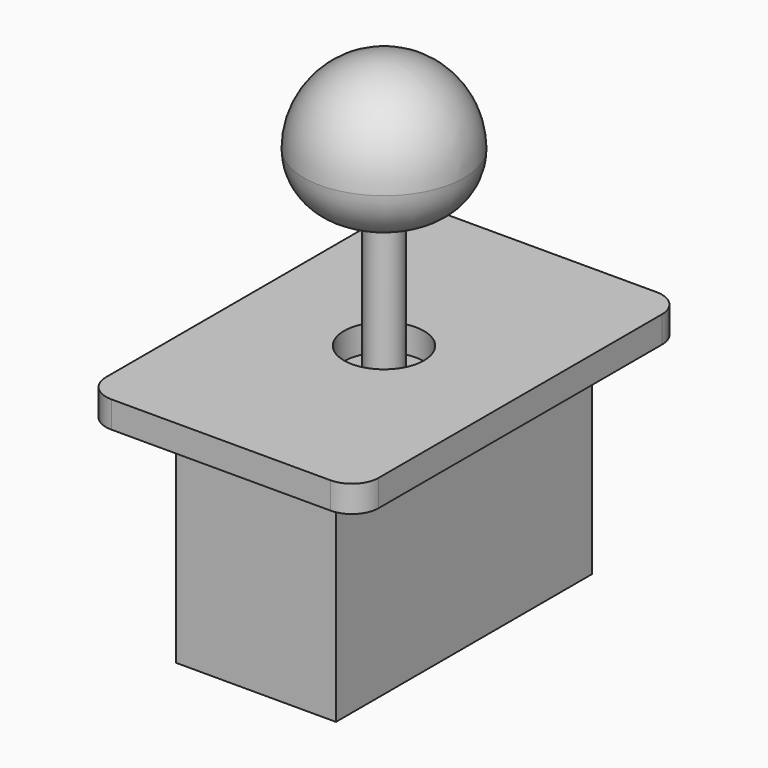
from build123d import *

# Parameters (mm, degrees)
F0_R     = 9.525
F1_DEPTH = 6.35
F2_R     = 4.1191118401
F3_DEPTH = 35
F4_R     = 19.05
F5_DEPTH = 31.75
F6_R     = 19.05
F7_R     = 12.69999
F8_W     = 38.1
F8_H     = 76.2
F8_R     = 9.525
F9_DEPTH = 50.8


# Not quite as in the source:
# - a fillet or chamfer is up to 0.001 mm smaller than in the source, because OpenCascade refuses the exact size


with BuildPart() as f1:
    # F0 (on Top) → F1 (new body)
    with BuildSketch(Plane.XY):
        with BuildLine():
            Line((26.095, 48.505), (-26.095, 48.505))
            ThreePointArc((-26.095, 48.505), (-30.5851280605, 46.6451280605), (-32.445, 42.155))
            Line((-32.445, 42.155), (-32.445, -42.155))
            ThreePointArc((-32.445, -42.155), (-30.5851280605, -46.6451280605), (-26.095, -48.505))
            Line((-26.095, -48.505), (26.095, -48.505))
            ThreePointArc((26.095, -48.505), (30.5851280605, -46.6451280605), (32.445, -42.155))
            Line((32.445, -42.155), (32.445, 42.155))
            ThreePointArc((32.445, 42.155), (30.5851280605, 46.6451280605), (26.095, 48.505))
        make_face()
        Circle(F0_R, mode=Mode.SUBTRACT)
    extrude(amount=-F1_DEPTH)


with BuildPart() as f3:
    # F2 (on face) → F3 (new body)
    with BuildSketch(Plane(origin=(0, 0, -6.35), x_dir=(1, 0, 0), z_dir=(0, 0, -1))):
        Circle(F2_R)
    extrude(amount=-F3_DEPTH)

    # F4 (on face) → F5 (join)
    with BuildSketch(Plane.XY.offset(28.65)):
        Circle(F4_R)
    extrude(amount=F5_DEPTH)

    # F6
    f6_edges = [f3.edges().sort_by_distance(p)[0] for p in [
        (-19.05, 0, 60.4),
    ]]
    fillet(f6_edges, radius=F6_R)

    # F7 (radius 12.7 in the source; OpenCascade refuses exactly that, so slightly less here)
    f7_edges = [f3.edges().sort_by_distance(p)[0] for p in [
        (-19.05, 0, 28.65),
    ]]
    fillet(f7_edges, radius=F7_R)


with BuildPart() as f9:
    # F8 (on face) → F9 (new body)
    with BuildSketch(Plane(origin=(0, 0, -6.35), x_dir=(1, 0, 0), z_dir=(0, 0, -1))):
        Rectangle(F8_W, F8_H)
        Circle(F8_R, mode=Mode.SUBTRACT)
        Circle(F8_R)
    extrude(amount=F9_DEPTH)


solid = Compound([f1.part, f3.part, f9.part])
